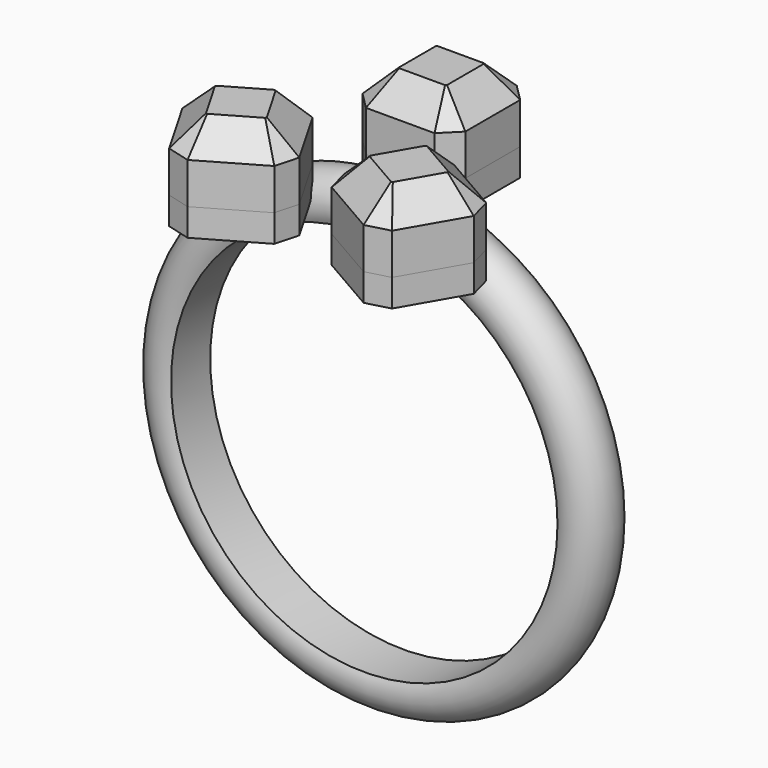
from build123d import *

# Parameters (mm, degrees)
F5_DEPTH  = 3.175
F6_SIZE   = 1.27
F6_2_SIZE = 1.27
F6_3_SIZE = 1.27
F7_DEPTH  = 1.27


with BuildPart() as f2:
    # F2: sweep along a path in F0
    with BuildLine(Plane.XZ) as f2_path:
        CenterArc((0, 0), 9.525, 0, 360)
    # F1 (on Top) → F2 (sweep)
    with BuildSketch(Plane.XY):
        with BuildLine():
            Line((-8.9527293057, 0), (-8.9527293057, 1.133757581))
            ThreePointArc((-8.9527293057, 1.133757581), (-10.795, 0), (-8.9527293057, -1.133757581))
            Line((-8.9527293057, -1.133757581), (-8.9527293057, 0))
        make_face()
    sweep(path=f2_path.line)

    # F4 (on offset) → F7 (join)
    with BuildSketch(Plane.XY.offset(10.795)):
        Polygon((2.625412817, -0.8479611432), (1.831662817, -2.2227764717), (1.037912817, -3.5975918002), (1.3284454812, -4.6818744645), (2.7032608097, -5.4756244645), (4.0780761382, -6.2693744645), (5.1623588025, -5.9788418002), (5.9561088025, -4.6040264717), (6.7498588025, -3.2292111432), (6.4593261382, -2.144928479), (5.0845108097, -1.351178479), (3.7096954812, -0.557428479), align=None)
        Polygon((-1.0379127641, -3.5975918002), (-1.8316627641, -2.2227764717), (-2.6254127641, -0.8479611432), (-3.7096954284, -0.557428479), (-5.0845107569, -1.351178479), (-6.4593260854, -2.144928479), (-6.7498587497, -3.2292111432), (-5.9561087497, -4.6040264717), (-5.1623587497, -5.9788418002), (-4.0780760854, -6.2693744645), (-2.7032607569, -5.4756244645), (-1.3284454284, -4.6818744645), align=None)
        Polygon((-1.5874999736, 0.9497565438), (2.64e-08, 0.9497565438), (1.5875000264, 0.9497565438), (2.3812500264, 1.7435065438), (2.3812500264, 3.3310065438), (2.3812500264, 4.9185065438), (1.5875000264, 5.7122565438), (2.64e-08, 5.7122565438), (-1.5874999736, 5.7122565438), (-2.3812499736, 4.9185065438), (-2.3812499736, 3.3310065438), (-2.3812499736, 1.7435065438), align=None)
    extrude(amount=-F7_DEPTH)


with BuildPart() as f5:
    # F4 (on offset) → F5 (new body)
    with BuildSketch(Plane.XY.offset(10.795)):
        Polygon((-1.5874999736, 0.9497565438), (2.64e-08, 0.9497565438), (1.5875000264, 0.9497565438), (2.3812500264, 1.7435065438), (2.3812500264, 3.3310065438), (2.3812500264, 4.9185065438), (1.5875000264, 5.7122565438), (2.64e-08, 5.7122565438), (-1.5874999736, 5.7122565438), (-2.3812499736, 4.9185065438), (-2.3812499736, 3.3310065438), (-2.3812499736, 1.7435065438), align=None)
    extrude(amount=F5_DEPTH)

    # F6
    f6_edges = [f5.edges().sort_by_distance(p)[0] for p in [
        (-1.984375, 1.346632, 13.97),
        (0, 0.949757, 13.97),
        (1.984375, 1.346632, 13.97),
        (2.38125, 3.331007, 13.97),
        (1.984375, 5.315382, 13.97),
        (0, 5.712257, 13.97),
        (-1.984375, 5.315382, 13.97),
        (-2.38125, 3.331007, 13.97),
    ]]
    chamfer(f6_edges, length=F6_SIZE)


with BuildPart() as f5b:
    # F4 (on offset) → F5, piece 2 (new body)
    with BuildSketch(Plane.XY.offset(10.795)):
        Polygon((-1.0379127641, -3.5975918002), (-1.8316627641, -2.2227764717), (-2.6254127641, -0.8479611432), (-3.7096954284, -0.557428479), (-5.0845107569, -1.351178479), (-6.4593260854, -2.144928479), (-6.7498587497, -3.2292111432), (-5.9561087497, -4.6040264717), (-5.1623587497, -5.9788418002), (-4.0780760854, -6.2693744645), (-2.7032607569, -5.4756244645), (-1.3284454284, -4.6818744645), align=None)
    extrude(amount=F5_DEPTH)

    # F6#2
    f6_2_edges = [f5b.edges().sort_by_distance(p)[0] for p in [
        (-1.831663, -2.222776, 13.97),
        (-3.167554, -0.702695, 13.97),
        (-5.084511, -1.351178, 13.97),
        (-6.604592, -2.68707, 13.97),
        (-5.956109, -4.604026, 13.97),
        (-4.620217, -6.124108, 13.97),
        (-2.703261, -5.475624, 13.97),
        (-1.183179, -4.139733, 13.97),
    ]]
    chamfer(f6_2_edges, length=F6_2_SIZE)


with BuildPart() as f5c:
    # F4 (on offset) → F5, piece 3 (new body)
    with BuildSketch(Plane.XY.offset(10.795)):
        Polygon((2.625412817, -0.8479611432), (1.831662817, -2.2227764717), (1.037912817, -3.5975918002), (1.3284454812, -4.6818744645), (2.7032608097, -5.4756244645), (4.0780761382, -6.2693744645), (5.1623588025, -5.9788418002), (5.9561088025, -4.6040264717), (6.7498588025, -3.2292111432), (6.4593261382, -2.144928479), (5.0845108097, -1.351178479), (3.7096954812, -0.557428479), align=None)
    extrude(amount=F5_DEPTH)

    # F6#3
    f6_3_edges = [f5c.edges().sort_by_distance(p)[0] for p in [
        (5.084511, -1.351178, 13.97),
        (3.167554, -0.702695, 13.97),
        (1.831663, -2.222776, 13.97),
        (1.183179, -4.139733, 13.97),
        (2.703261, -5.475624, 13.97),
        (4.620217, -6.124108, 13.97),
        (5.956109, -4.604026, 13.97),
        (6.604592, -2.68707, 13.97),
    ]]
    chamfer(f6_3_edges, length=F6_3_SIZE)


solid = Compound([f2.part, f5.part, f5b.part, f5c.part])
